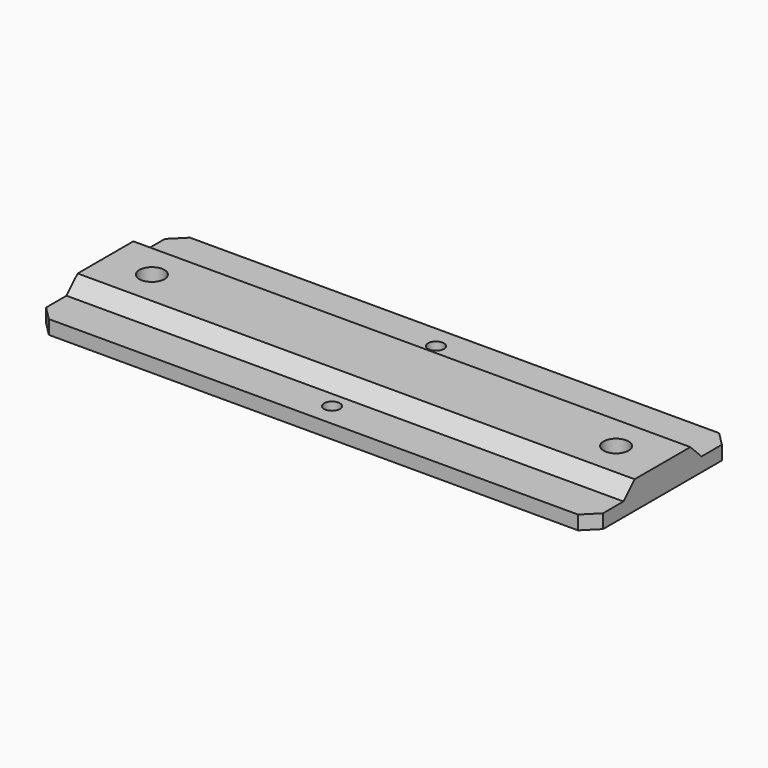
from build123d import *

# Parameters (mm, degrees)
F0_R     = 1.7
F1_DEPTH = 3
F0_R_2   = 4.7
F0_R_3   = 2.7
F2_DEPTH = 6
F3_DEPTH = 2
F4_SIZE  = 2.99999
F5_START = 2
F5_DEPTH = 0.3


# Not quite as in the source:
# - a fillet or chamfer is up to 0.001 mm smaller than in the source, because OpenCascade refuses the exact size


with BuildPart() as f1:
    # F0 (on Top) → F1 (new body)
    with BuildSketch(Plane.XY):
        Polygon((12.5, 19), (-12.5, 19), (-60, 19), (-60, 7.5), (-12.5, 7.5), (12.5, 7.5), (60, 7.5), (60, 19), align=None)
        with Locations((0, 14)):
            Circle(F0_R, mode=Mode.SUBTRACT)
    extrude(amount=F1_DEPTH)



with BuildPart() as f1b:
    # F0 (on Top) → F1, piece 2 (new body)
    with BuildSketch(Plane.XY):
        Polygon((-12.5, -7.5), (-60, -7.5), (-60, -19), (-8.9196664095, -19), (8.9196664095, -19), (16.0803335905, -19), (60, -19), (60, -7.5), (12.5, -7.5), align=None)
        with Locations((0, -14)):
            Circle(F0_R, mode=Mode.SUBTRACT)
    extrude(amount=F1_DEPTH)


with BuildPart() as f1_1:
    add(f1.part)

    add(f1b.part)  # F2 merges F1b
    # F0 (on Top) → F2 (join)
    with BuildSketch(Plane.XY):
        Polygon((-12.5, 7.5), (-60, 7.5), (-60, -7.5), (-12.5, -7.5), (12.5, -7.5), (60, -7.5), (60, 7.5), (12.5, 7.5), align=None)
        with Locations((-50, 0)):
            Circle(F0_R_2, mode=Mode.SUBTRACT)
        with Locations((50, 0)):
            Circle(F0_R_2, mode=Mode.SUBTRACT)
        with Locations((-50, 0)):
            Circle(F0_R_2)
        with Locations((-50, 0)):
            Circle(F0_R_3, mode=Mode.SUBTRACT)
        with Locations((50, 0)):
            Circle(F0_R_2)
        with Locations((50, 0)):
            Circle(F0_R_3, mode=Mode.SUBTRACT)
    extrude(amount=F2_DEPTH)

    # F0 (on Top) → F3 (cut)
    with BuildSketch(Plane.XY):
        with Locations((-50, 0)):
            Circle(F0_R_2)
        with Locations((-50, 0)):
            Circle(F0_R_3, mode=Mode.SUBTRACT)
        with Locations((50, 0)):
            Circle(F0_R_2)
        with Locations((50, 0)):
            Circle(F0_R_3, mode=Mode.SUBTRACT)
    extrude(amount=F3_DEPTH, mode=Mode.SUBTRACT)

    # F4 (size 3 in the source; OpenCascade refuses exactly that, so slightly less here)
    f4_edges = [f1_1.edges().sort_by_distance(p)[0] for p in [
        (0, 7.5, 3),
        (0, -7.5, 3),
        (-60, -19, 1.5),
        (-60, 19, 1.5),
        (60, -19, 1.5),
        (60, 19, 1.5),
    ]]
    chamfer(f4_edges, length=F4_SIZE)

    # F0 (on Top) → F5 (join)
    with BuildSketch(Plane.XY.offset(F5_START)):
        with Locations((-50, 0)):
            Circle(F0_R_3)
        with Locations((50, 0)):
            Circle(F0_R_3)
    extrude(amount=F5_DEPTH)


solid = f1_1.part
